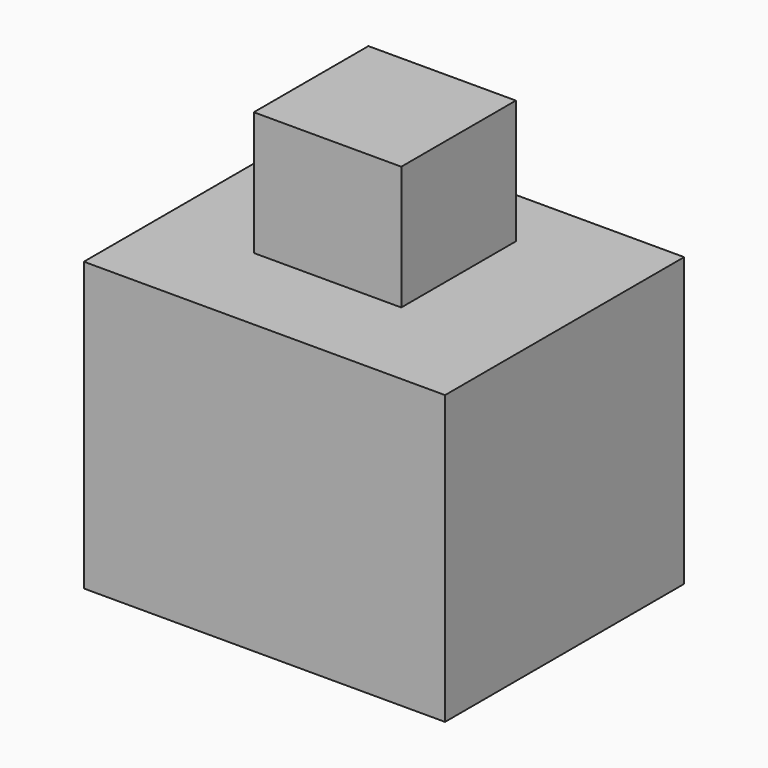
from build123d import *

# Parameters (mm, degrees)
F0_W     = 101.6
F0_H     = 105.0883368849
F1_DEPTH = 101.1590287089
F2_W     = 105.0883368849
F2_H     = 101.1590287089
F3_DEPTH = 25.4
F6_W     = 51.8510639668
F6_H     = 50.3680855036
F7_DEPTH = 43.5765609145


# Not quite as in the source:
# - the program builds the solid bodies; features that only make, move or delete a surface that nothing else refers to are left out


with BuildPart() as f1:
    # F0 (on Top) → F1 (new body)
    with BuildSketch(Plane.XY):
        with Locations((-2.9358975589, -0.3588087857)):
            Rectangle(F0_W, F0_H)
    extrude(amount=F1_DEPTH)

    # F2 (on face) → F3 (join)
    with BuildSketch(Plane.YZ.offset(47.8641024411)):
        with Locations((-0.3588087857, 50.5795143545)):
            Rectangle(F2_W, F2_H)
    extrude(amount=F3_DEPTH)

    # F6 (on face) → F7 (join)
    with BuildSketch(Plane.XY.offset(101.1590287089)):
        with Locations((5.4090619087, 5.453877151)):
            Rectangle(F6_W, F6_H)
    extrude(amount=F7_DEPTH)


solid = f1.part
